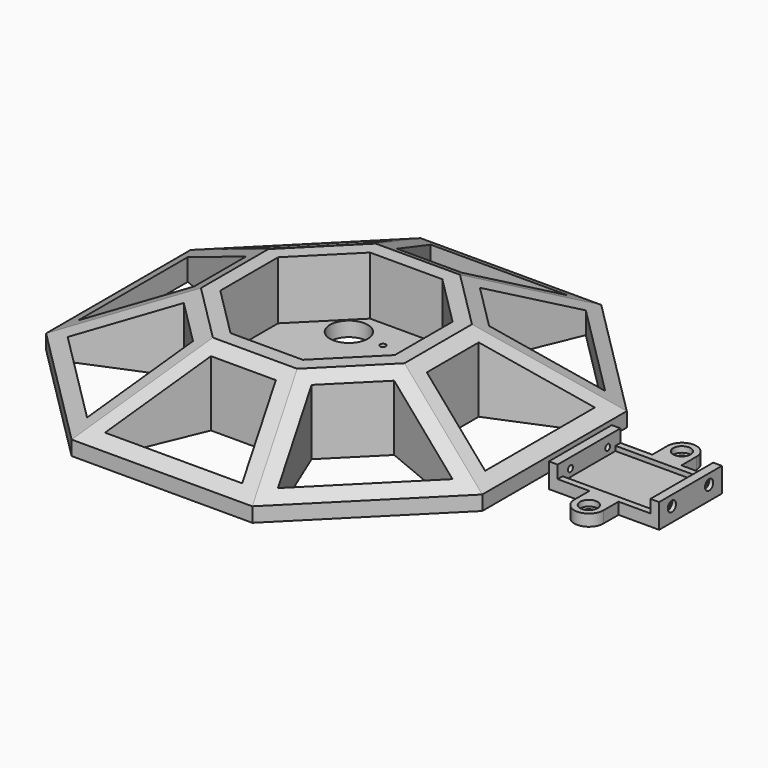
from build123d import *

# Parameters (mm, degrees)
F2_DEPTH  = 25
F3_SIZE2  = 40
F3_SIZE   = 20
F5_DEPTH  = 20
F6_R      = 1
F7_DEPTH  = 25
F9_DEPTH  = 25
F6_R_2    = 1.75
F10_DEPTH = 1.4
F11_W     = 3
F11_H     = 27
F12_DEPTH = 4
F13_DEPTH = 8.4
F14_W     = 31.9
F14_H     = 22.7
F15_DEPTH = 1.6
F16_R     = 1.05
F17_DEPTH = 5
F16_R_2   = 1.775
F18_DEPTH = 1.4
F19_R     = 1.05
F20_DEPTH = 4
F19_R_2   = 1.775
F21_DEPTH = 1.4
F22_R     = 1.5
F23_DEPTH = 25
F22_R_2   = 3
F24_DEPTH = 2
F25_R     = 1
F26_DEPTH = 25
F27_R     = 6.5
F28_DEPTH = 25


# Not quite as in the source:
# - a feature names something its author has since deleted; it is built from what else it names


with BuildPart() as f2:
    # F1 (on offset) → F2 (new body)
    with BuildSketch(Plane.XY):
        Polygon((75, -31.066017178), (75, 31.066017178), (31.066017178, 75), (-31.066017178, 75), (-75, 31.066017178), (-75, -31.066017178), (-31.066017178, -75), (31.066017178, -75), align=None)
    extrude(amount=F2_DEPTH)

    # F3
    f3_edges = [f2.edges().sort_by_distance(p)[0] for p in [
        (-75, 0, 25),
        (75, 0, 25),
        (53.033009, 53.033009, 25),
        (0, 75, 25),
        (-53.033009, 53.033009, 25),
        (-53.033009, -53.033009, 25),
        (0, -75, 25),
        (53.033009, -53.033009, 25),
    ]]
    chamfer(f3_edges, length=F3_SIZE, length2=F3_SIZE2)

    # F4 (on face) → F5 (cut)
    with BuildSketch(Plane.XY.offset(25)):
        Polygon((-30, -12.4264068712), (-12.4264068712, -30), (12.4264068712, -30), (30, -12.4264068712), (30, 12.4264068712), (12.4264068712, 30), (-12.4264068712, 30), (-30, 12.4264068712), align=None)
    extrude(amount=-F5_DEPTH, mode=Mode.SUBTRACT)

    # F6 (on face) → F7 (cut)
    with BuildSketch(Plane.XY.offset(5)):
        with Locations((8, 0)):
            Circle(F6_R)
        with Locations((0, 8)):
            Circle(F6_R)
        with Locations((-8, 0)):
            Circle(F6_R)
        with Locations((0, -8)):
            Circle(F6_R)
    extrude(amount=-F7_DEPTH, mode=Mode.SUBTRACT)

    # F8 (on face) → F9 (cut)
    with BuildSketch(Plane(origin=(0, 0, 0), x_dir=(1, 0, 0), z_dir=(0, 0, -1))):
        Polygon((-66.1731656763, 32.8217836898), (-36.1731656763, 20.3953768186), (-20.3953768186, 36.1731656763), (-32.8217836898, 66.1731656763), align=None)
        Polygon((-11.1565814935, 40), (11.1565814935, 40), (23.5829883647, 70), (-23.5829883647, 70), align=None)
        Polygon((32.8217836898, 66.1731656763), (20.3953768186, 36.1731656763), (36.1731656763, 20.3953768186), (66.1731656763, 32.8217836898), align=None)
        Polygon((70, -23.5829883647), (70, 23.5829883647), (40, 11.1565814935), (40, -11.1565814935), align=None)
        Polygon((32.8217836898, -66.1731656763), (66.1731656763, -32.8217836898), (36.1731656763, -20.3953768186), (20.3953768186, -36.1731656763), align=None)
        Polygon((-23.5829883647, -70), (23.5829883647, -70), (11.1565814935, -40), (-11.1565814935, -40), align=None)
        Polygon((-66.1731656763, -32.8217836898), (-32.8217836898, -66.1731656763), (-20.3953768186, -36.1731656763), (-36.1731656763, -20.3953768186), align=None)
        Polygon((-70, -23.5829883647), (-40, -11.1565814935), (-40, 11.1565814935), (-70, 23.5829883647), align=None)
    extrude(amount=-F9_DEPTH, mode=Mode.SUBTRACT)

    # F6 (on face) → F10 (cut)
    with BuildSketch(Plane.XY.offset(5)):
        with Locations((-8, 0)):
            Circle(F6_R_2)
        with Locations((-8, 0)):
            Circle(F6_R, mode=Mode.SUBTRACT)
        with Locations((0, 8)):
            Circle(F6_R_2)
        with Locations((0, 8)):
            Circle(F6_R, mode=Mode.SUBTRACT)
        with Locations((8, 0)):
            Circle(F6_R_2)
        with Locations((8, 0)):
            Circle(F6_R, mode=Mode.SUBTRACT)
        with Locations((0, -8)):
            Circle(F6_R_2)
        with Locations((0, -8)):
            Circle(F6_R, mode=Mode.SUBTRACT)
    extrude(amount=-F10_DEPTH, mode=Mode.SUBTRACT)

    # F25 (on face) → F26 (cut)
    with BuildSketch(Plane.XY.offset(5)):
        with Locations((0, 20)):
            Circle(F25_R)
        with Locations((0, -20)):
            Circle(F25_R)
    extrude(amount=-F26_DEPTH, mode=Mode.SUBTRACT)

    # F27 (on face) → F28 (cut)
    with BuildSketch(Plane.XY.offset(5)):
        with Locations((-12.0903318748, 20.4435605556)):
            Circle(F27_R)
    extrude(amount=-F28_DEPTH, mode=Mode.SUBTRACT)


with BuildPart() as f12:
    # F11 (on offset) → F12 (new body)
    with BuildSketch(Plane.XY):
        with Locations((82.5181498528, 3.5604816154)):
            Rectangle(F11_W, F11_H)
        Polygon((94.9681498528, 17.0604816154), (84.0181498528, 17.0604816154), (84.0181498528, -9.9395183846), (94.9681498528, -9.9395183846), (104.9681498528, -9.9395183846), (115.9181498528, -9.9395183846), (115.9181498528, 17.0604816154), (104.9681498528, 17.0604816154), align=None)
        with BuildLine():
            Line((94.9681498528, 23.5604816154), (94.9681498528, 17.0604816154))
            Line((94.9681498528, 17.0604816154), (104.9681498528, 17.0604816154))
            Line((104.9681498528, 17.0604816154), (104.9681498528, 23.5604816154))
            ThreePointArc((104.9681498528, 23.5604816154), (99.9681498528, 28.5604816154), (94.9681498528, 23.5604816154))
        make_face()
        with BuildLine():
            Line((104.9681498528, -9.9395183846), (94.9681498528, -9.9395183846))
            Line((94.9681498528, -9.9395183846), (94.9681498528, -16.4395183846))
            ThreePointArc((94.9681498528, -16.4395183846), (99.9681498528, -21.4395183846), (104.9681498528, -16.4395183846))
            Line((104.9681498528, -16.4395183846), (104.9681498528, -9.9395183846))
        make_face()
        with Locations((117.4181498528, 3.5604816154)):
            Rectangle(F11_W, F11_H)
    extrude(amount=F12_DEPTH)

    # F11 (on offset) → F13 (join)
    with BuildSketch(Plane.XY):
        with Locations((82.5181498528, 3.5604816154)):
            Rectangle(F11_W, F11_H)
        with Locations((117.4181498528, 3.5604816154)):
            Rectangle(F11_W, F11_H)
    extrude(amount=F13_DEPTH)

    # F14 (on face) → F15 (cut)
    with BuildSketch(Plane.XY.offset(4)):
        with Locations((99.9681498528, 3.5604816154)):
            Rectangle(F14_W, F14_H)
    extrude(amount=-F15_DEPTH, mode=Mode.SUBTRACT)

    # F16 (on face) → F17 (cut)
    with BuildSketch(Plane.YZ.offset(118.9181498528)):
        with Locations((11.5604816154, 4.9)):
            Circle(F16_R)
        with Locations((-4.4395183846, 4.9)):
            Circle(F16_R)
    extrude(amount=-F17_DEPTH, mode=Mode.SUBTRACT)

    # F16 (on face) → F18 (cut)
    with BuildSketch(Plane.YZ.offset(118.9181498528)):
        with Locations((-4.4395183846, 4.9)):
            Circle(F16_R_2)
        with Locations((-4.4395183846, 4.9)):
            Circle(F16_R, mode=Mode.SUBTRACT)
        with Locations((11.5604816154, 4.9)):
            Circle(F16_R_2)
        with Locations((11.5604816154, 4.9)):
            Circle(F16_R, mode=Mode.SUBTRACT)
    extrude(amount=-F18_DEPTH, mode=Mode.SUBTRACT)

    # F19 (on face) → F20 (cut)
    with BuildSketch(Plane(origin=(81.0181498528, 0, 0), x_dir=(0, -1, 0), z_dir=(-1, 0, 0))):
        with Locations((4.4243399079, 4.9480630373)):
            Circle(F19_R)
        with Locations((-11.5753707892, 4.8518465555)):
            Circle(F19_R)
    extrude(amount=-F20_DEPTH, mode=Mode.SUBTRACT)

    # F19 (on face) → F21 (cut)
    with BuildSketch(Plane(origin=(81.0181498528, 0, 0), x_dir=(0, -1, 0), z_dir=(-1, 0, 0))):
        with Locations((-11.5753707892, 4.8518465555)):
            Circle(F19_R_2)
        with Locations((-11.5753707892, 4.8518465555)):
            Circle(F19_R, mode=Mode.SUBTRACT)
        with Locations((4.4243399079, 4.9480630373)):
            Circle(F19_R_2)
        with Locations((4.4243399079, 4.9480630373)):
            Circle(F19_R, mode=Mode.SUBTRACT)
    extrude(amount=-F21_DEPTH, mode=Mode.SUBTRACT)

    # F22 (on face) → F23 (cut)
    with BuildSketch(Plane.XY.offset(4)):
        with Locations((99.9681498528, 23.5604816154)):
            Circle(F22_R)
        with Locations((99.9681498528, -16.4395183846)):
            Circle(F22_R)
    extrude(amount=-F23_DEPTH, mode=Mode.SUBTRACT)

    # F22 (on face) → F24 (cut)
    with BuildSketch(Plane.XY.offset(4)):
        with Locations((99.9681498528, -16.4395183846)):
            Circle(F22_R_2)
        with Locations((99.9681498528, -16.4395183846)):
            Circle(F22_R, mode=Mode.SUBTRACT)
        with Locations((99.9681498528, 23.5604816154)):
            Circle(F22_R_2)
        with Locations((99.9681498528, 23.5604816154)):
            Circle(F22_R, mode=Mode.SUBTRACT)
    extrude(amount=-F24_DEPTH, mode=Mode.SUBTRACT)


solid = Compound([f2.part, f12.part])
